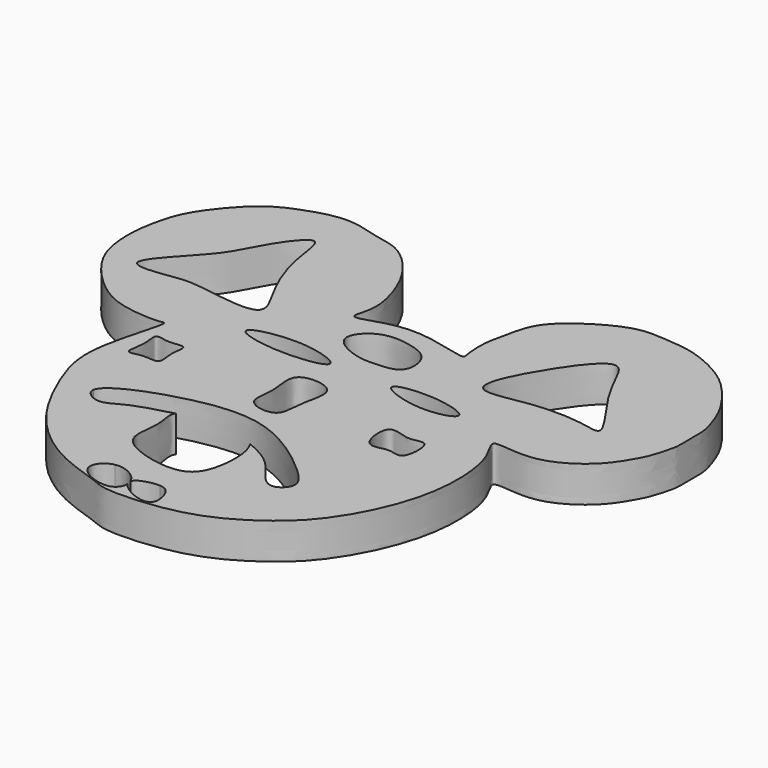
from build123d import *

# Parameters (mm, degrees)
F1_DEPTH = 5


with BuildPart() as f1:
    # F0 (on Top) → F1 (new body)
    with BuildSketch(Plane.XY):
        with BuildLine():
            add(Edge.make_bspline(
                [(-43.649811, 53.334028), (-43.292363, 52.997825), (-39.822842, 54.44877), (-34.65125, 54.987145), (-28.253329, 52.836346), (-28.551042, 53.985154), (-28.889519, 57.038411), (-27.946027, 60.843134), (-27.020346, 65.281317), (-19.624599, 69.90776), (-16.556934, 70.297191), (-15.257369, 70.278093), (-12.897785, 70.107045), (-10.245593, 69.809275), (-7.437441, 68.852641), (-3.537279, 66.793835), (-0.647238, 63.424451), (1.280854, 60.600981), (2.582232, 56.875783), (2.761459, 55.275956), (2.716647, 52.033555), (2.752842, 51.097927), (1.874652, 47.754197), (0.929136, 46.179015), (-1.000734, 42.66303), (-7.346991, 38.368623), (-14.618343, 40.40914), (-11.079555, 36.287133), (-10.356761, 25.496922), (-15.721139, 14.620493), (-21.060865, 9.652727), (-28.848527, 5.067558), (-39.497963, 4.555195), (-41.4943, 5.771558), (-48.228918, 7.61443), (-55.429395, 13.398743), (-59.798102, 22.501411), (-61.77129, 29.491871), (-58.137182, 39.659291), (-59.429782, 39.063491), (-64.489483, 39.220528), (-69.021568, 41.337084), (-73.858812, 46.713847), (-74.725789, 50.882551), (-74.784267, 53.884193), (-74.39706, 56.658133), (-73.529803, 60.065777), (-71.602149, 63.157501), (-67.882155, 67.517101), (-63.36318, 69.515338), (-58.08694, 71.010864), (-53.453141, 69.31463), (-50.042887, 68.993651), (-46.121614, 65.35359), (-43.74203, 60.400591), (-42.879793, 55.810327), (-43.938126, 53.605206), (-43.649811, 53.334028)],
                knots=[0, 0, 0, 0, 0.015736, 0.037555, 0.05799, 0.064119, 0.079088, 0.096349, 0.114508, 0.139556, 0.154423, 0.163919, 0.177014, 0.19119, 0.206015, 0.224111, 0.242215, 0.258518, 0.275167, 0.286748, 0.301728, 0.310812, 0.326303, 0.338319, 0.355049, 0.379196, 0.398738, 0.413429, 0.441979, 0.471912, 0.494897, 0.521172, 0.548433, 0.561508, 0.583402, 0.609911, 0.636785, 0.661473, 0.687328, 0.693349, 0.712245, 0.73228, 0.755069, 0.772714, 0.787396, 0.801812, 0.817748, 0.834339, 0.854739, 0.874047, 0.893994, 0.912787, 0.92852, 0.947863, 0.96839, 0.987307, 1, 1, 1, 1], degree=3))
        make_face()
        with BuildLine():
            add(Edge.make_bspline(
                [(-42.126976, 9.954481), (-43.347124, 9.731022), (-45.610035, 7.111511), (-39.382703, 4.648006), (-38.254226, 6.545566), (-38.273395, 7.264431)],
                knots=[0, 0, 0, 0, 0.22846, 0.521383, 0.678997, 0.678997, 0.678997, 0.678997], degree=3))
            add(Edge.make_bspline(
                [(-38.425617, 7.971691), (-38.928385, 9.194327), (-40.68689, 10.218221), (-42.126976, 9.954481)],
                knots=[0.730359, 0.730359, 0.730359, 0.730359, 1, 1, 1, 1], degree=3))
            add(Edge.make_bspline(
                [(-35.253022, 9.161365), (-36.364727, 9.255924), (-38.195894, 8.747816), (-38.425617, 7.971691)],
                knots=[0, 0, 0, 0, 0.224931, 0.224931, 0.224931, 0.224931], degree=3))
            add(Edge.make_bspline(
                [(-38.273395, 7.264431), (-37.891488, 6.654878), (-35.806584, 5.251625), (-32.951597, 5.05062), (-33.508171, 8.203759), (-34.402587, 9.089029), (-35.253022, 9.161365)],
                knots=[0.288753, 0.288753, 0.288753, 0.288753, 0.447382, 0.641597, 0.827932, 1, 1, 1, 1], degree=3))
        make_face(mode=Mode.SUBTRACT)
        with BuildLine():
            add(Edge.make_bspline(
                [(-44.50608, 23.437455), (-45.037679, 22.792169), (-43.987219, 20.428035), (-45.538021, 15.670228), (-40.761173, 13.319581), (-34.644931, 12.641614), (-32.705574, 16.832895), (-32.792823, 21.568026), (-33.799011, 22.908712)],
                knots=[0, 0, 0, 0, 0.097912, 0.217829, 0.340393, 0.475778, 0.590548, 0.731052, 0.731052, 0.731052, 0.731052], degree=3))
            add(Edge.make_bspline(
                [(-44.50608, 23.437455), (-46.564068, 22.898688), (-50.176232, 21.940677), (-52.809346, 19.81571), (-55.097751, 21.398889), (-54.948773, 22.247782)],
                knots=[0.794307, 0.794307, 0.794307, 0.794307, 0.881117, 0.943575, 1, 1, 1, 1], degree=3))
            add(Edge.make_bspline(
                [(-54.948773, 22.247782), (-54.611212, 24.17125), (-42.033105, 28.736281), (-33.160771, 27.06623), (-26.203087, 21.761863), (-23.026122, 18.300331), (-26.491975, 15.455811), (-29.360876, 20.949503), (-32.288893, 22.249181), (-33.799011, 22.908712)],
                knots=[0, 0, 0, 0, 0.12785, 0.240782, 0.344567, 0.413243, 0.468919, 0.548688, 0.627988, 0.627988, 0.627988, 0.627988], degree=3))
        make_face(mode=Mode.SUBTRACT)
        with BuildLine():
            add(Edge.make_bspline(
                [(-55.610489, 36.127314), (-54.77805, 36.094803), (-53.05274, 36.697454), (-53.932634, 34.126448), (-52.98971, 31.296113), (-55.730853, 32.067967), (-58.224198, 30.994664), (-57.106383, 34.006088), (-58.047741, 36.880978), (-56.415726, 36.158763), (-55.610489, 36.127314)],
                knots=[0, 0, 0, 0, 0.122043, 0.244084, 0.374007, 0.500175, 0.61823, 0.752022, 0.881945, 1, 1, 1, 1], degree=3))
        make_face(mode=Mode.SUBTRACT)
        with BuildLine():
            add(Edge.make_bspline(
                [(-39.483149, 38.374476), (-40.357519, 37.588466), (-39.273524, 34.353238), (-40.423192, 30.914129), (-37.929006, 29.820239), (-35.292838, 30.219415), (-35.591157, 34.034539), (-33.740943, 38.879404), (-38.580205, 39.186171), (-39.483149, 38.374476)],
                knots=[0, 0, 0, 0, 0.157499, 0.301116, 0.416458, 0.529632, 0.677429, 0.837354, 1, 1, 1, 1], degree=3))
        make_face(mode=Mode.SUBTRACT)
        with BuildLine():
            add(Edge.make_bspline(
                [(-24.148954, 34.937639), (-23.553392, 35.530725), (-21.113165, 34.026179), (-18.39901, 35.82361), (-18.587825, 30.013124), (-21.14202, 31.631845), (-24.342386, 29.787889), (-24.818209, 34.271167), (-24.148954, 34.937639)],
                knots=[0, 0, 0, 0, 0.173166, 0.317324, 0.504652, 0.644233, 0.805407, 1, 1, 1, 1], degree=3))
        make_face(mode=Mode.SUBTRACT)
        with BuildLine():
            add(Edge.make_bspline(
                [(-44.38065, 44.78164), (-47.44328, 44.931964), (-53.671567, 43.440959), (-45.209748, 41.316753), (-35.747098, 42.627447), (-41.459663, 44.638269), (-44.38065, 44.78164)],
                knots=[0, 0, 0, 0, 0.256715, 0.497559, 0.755158, 1, 1, 1, 1], degree=3))
        make_face(mode=Mode.SUBTRACT)
        with BuildLine():
            add(Edge.make_bspline(
                [(-41.201636, 48.684984), (-41.425831, 49.721696), (-39.305107, 52.376651), (-34.86352, 52.073246), (-31.334666, 50.712269), (-31.03853, 46.374281), (-34.531637, 45.97771), (-37.742322, 45.900303), (-40.960488, 47.569879), (-41.201636, 48.684984)],
                knots=[0, 0, 0, 0, 0.142121, 0.300485, 0.442053, 0.577038, 0.703822, 0.847132, 1, 1, 1, 1], degree=3))
        make_face(mode=Mode.SUBTRACT)
        with BuildLine():
            add(Edge.make_bspline(
                [(-69.887154, 48.420612), (-69.471202, 47.565747), (-63.935981, 48.467041), (-61.514169, 48.573446), (-50.26868, 46.354264), (-54.786102, 53.079083), (-57.134242, 59.440977), (-57.49168, 66.538033), (-62.291351, 59.894806), (-63.692965, 55.619585), (-70.418239, 49.512097), (-69.887154, 48.420612)],
                knots=[0, 0, 0, 0, 0.103662, 0.194565, 0.324223, 0.423433, 0.55477, 0.649062, 0.752638, 0.867645, 1, 1, 1, 1], degree=3))
        make_face(mode=Mode.SUBTRACT)
        with BuildLine():
            add(Edge.make_bspline(
                [(-25.369579, 43.797866), (-27.765657, 43.940669), (-32.751153, 43.144695), (-24.649312, 40.208746), (-17.983024, 42.257262), (-22.851688, 43.647803), (-25.369579, 43.797866)],
                knots=[0, 0, 0, 0, 0.243162, 0.510738, 0.744476, 1, 1, 1, 1], degree=3))
        make_face(mode=Mode.SUBTRACT)
        with BuildLine():
            add(Edge.make_bspline(
                [(-22.298275, 48.949357), (-21.560718, 47.998039), (-15.951525, 49.536689), (-9.362587, 49.46283), (-4.221146, 47.852552), (-11.691538, 56.534343), (-13.865172, 64.565887), (-19.772076, 56.847302), (-23.171435, 50.075579), (-22.298275, 48.949357)],
                knots=[0, 0, 0, 0, 0.134638, 0.290525, 0.379049, 0.547769, 0.687945, 0.840608, 1, 1, 1, 1], degree=3))
        make_face(mode=Mode.SUBTRACT)
    extrude(amount=F1_DEPTH)


solid = f1.part
